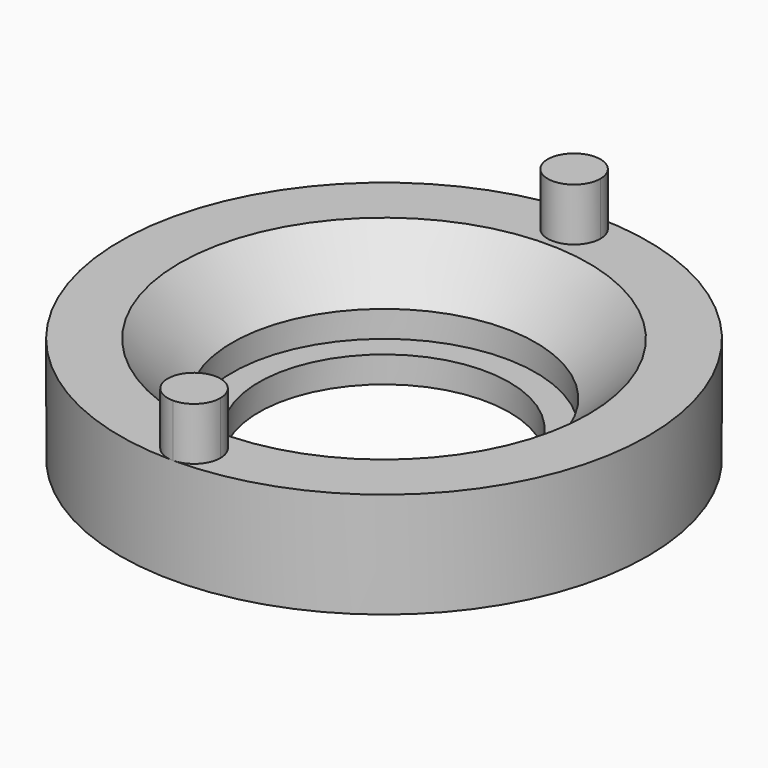
from build123d import *

# Parameters (mm, degrees)
F0_R     = 10
F0_R_2   = 5.75
F1_DEPTH = 4
F0_R_3   = 4.75
F2_DEPTH = 1
F3_SIZE  = 2
F5_DEPTH = 2


# Not quite as in the source:
# - a feature names something its author has since deleted; it is built from what else it names


with BuildPart() as f1:
    # F0 (on Top) → F1 (new body)
    with BuildSketch(Plane.XY):
        Circle(F0_R)
        Circle(F0_R_2, mode=Mode.SUBTRACT)
    extrude(amount=F1_DEPTH)

    # F0 (on Top) → F2 (join)
    with BuildSketch(Plane.XY):
        Circle(F0_R_2)
        Circle(F0_R_3, mode=Mode.SUBTRACT)
    extrude(amount=F2_DEPTH)

    # F3
    f3_edges = [f1.edges().sort_by_distance(p)[0] for p in [
        (-5.75, 0, 4),
    ]]
    chamfer(f3_edges, length=F3_SIZE)

    # F4 (on face) → F5 (join)
    with BuildSketch(Plane.XY.offset(4)):
        with BuildLine():
            ThreePointArc((4.5e-09, 10), (-0.7071067828, 8.2928932204), (1, 9))
            ThreePointArc((1, 9), (0.7071067828, 9.7071067796), (4.5e-09, 10))
        make_face()
        with BuildLine():
            ThreePointArc((1, -9), (-0.7071067792, -8.2928932169), (-5.5e-09, -10))
            ThreePointArc((-5.5e-09, -10), (0.7071067792, -9.7071067831), (1, -9))
        make_face()
    extrude(amount=F5_DEPTH)


solid = f1.part
